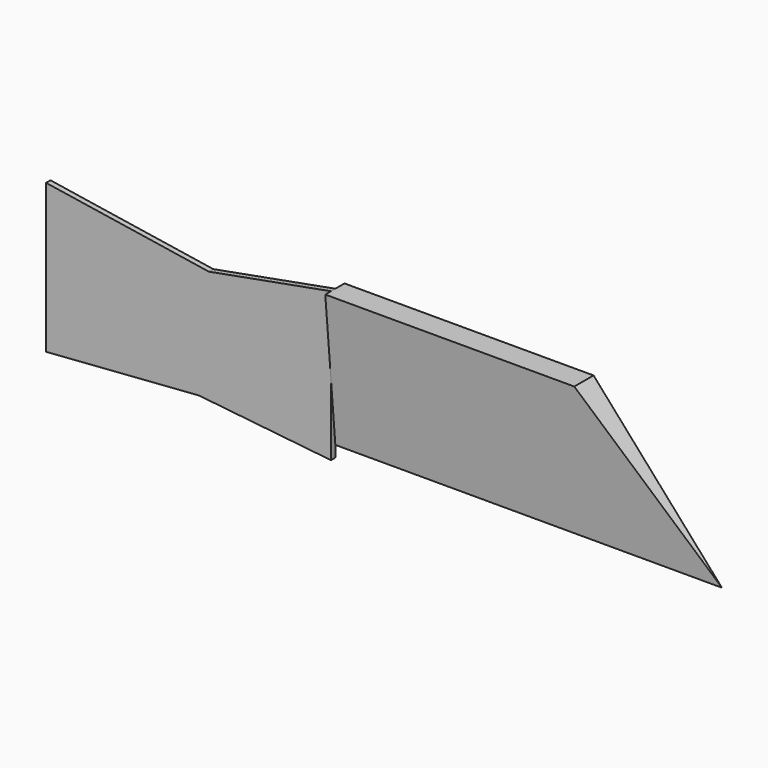
from build123d import *

# Parameters (mm, degrees)
F1_DEPTH    = 59.944
F2_T1_DEPTH = 133.9811516914
F4_DEPTH    = 0.762


# Not quite as in the source:
# - a fillet or chamfer that OpenCascade refuses, or shapes differently, is made with other operations: its cross-section is extruded or revolved along the edge and cut away or added


with BuildPart() as f1:
    # F0 (on Right) → F1 (new body)
    with BuildSketch(Plane.YZ):
        Polygon((1.5876128762, 10.7069341466), (0, 10.7069341466), (-1.7520430265, 10.7069341466), (0, -8.3708763123), align=None)
    extrude(amount=F1_DEPTH)

    # F2: chamfer of 25.4 on 1 edges, made by hand

    # F2_s2 → F2_t1 (cut)
    with BuildSketch(Plane.XZ.offset(-66.9083607706)):
        Polygon((59.944, -14.6930658534), (34.544, 10.7069341466), (59.944, 10.7069341466), align=None)
    extrude(amount=F2_T1_DEPTH, mode=Mode.SUBTRACT)

    # F3 (on Front) → F4 (join)
    with BuildSketch(Plane.XZ):
        Polygon((0, -9.9282488227), (0, 10.7069341466), (-16.936423257, 7.592190057), (-39.5183227956, 11.0962782055), (-39.5183227956, -9.5389056951), (-18.2991251349, -7.9815322533), align=None)
    extrude(amount=F4_DEPTH)


solid = f1.part
